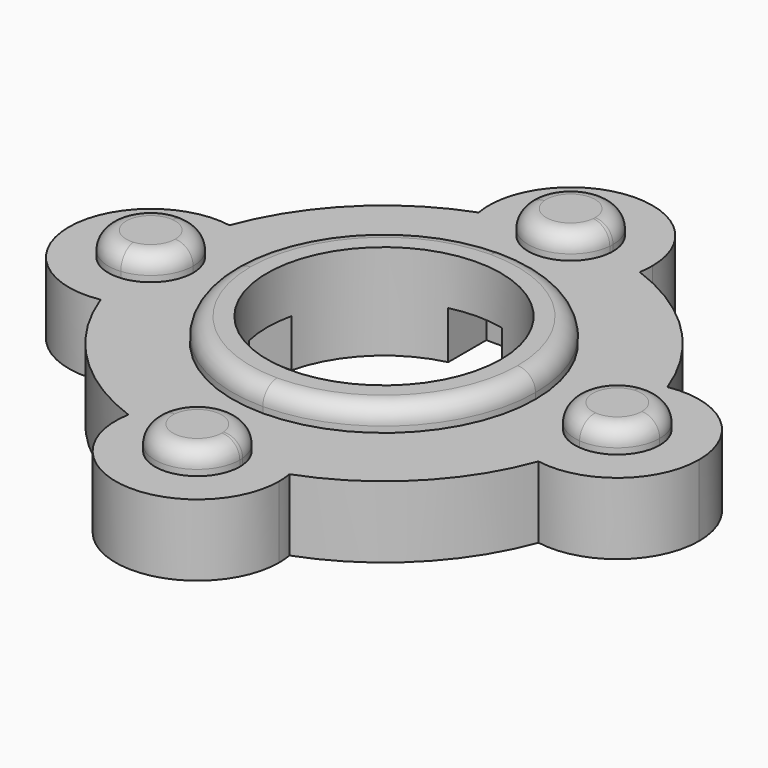
from build123d import *

# Parameters (mm, degrees)
F0_R     = 4.9
F1_DEPTH = 3
F2_DEPTH = 4
F4_DEPTH = 2
F5_R     = 0.75


with BuildPart() as f1:
    # F0 (on Top) → F1 (new body)
    with BuildSketch(Plane.XY):
        with BuildLine():
            ThreePointArc((-9.6173636364, -1.7706376495), (-9.779, 0), (-9.6173636364, 1.7706376495))
            ThreePointArc((-9.6173636364, 1.7706376495), (-11.557, 0), (-9.6173636364, -1.7706376495))
        make_face()
        with BuildLine():
            ThreePointArc((1.778, 9.779), (-0.080901975, 11.5551584587), (-1.7706376495, 9.6173636364))
            ThreePointArc((-1.7706376495, 9.6173636364), (0, 9.779), (1.7706376495, 9.6173636364))
            ThreePointArc((1.7706376495, 9.6173636364), (1.7761584587, 9.698098025), (1.778, 9.779))
        make_face()
        with BuildLine():
            ThreePointArc((-3.3758870855, -9.1778116883), (-2.201881727, -7.1503581719), (0, -6.35))
            ThreePointArc((0, -6.35), (-4.4901280605, -4.4901280605), (-6.35, 0))
            ThreePointArc((-6.35, 0), (-7.1503581719, -2.201881727), (-9.1778116883, -3.3758870855))
            ThreePointArc((-9.1778116883, -3.3758870855), (-6.9147972132, -6.9147972132), (-3.3758870855, -9.1778116883))
        make_face()
        with BuildLine():
            ThreePointArc((-8.001, 0), (-8.4658599742, 1.1987273555), (-9.6173636364, 1.7706376495))
            ThreePointArc((-9.6173636364, 1.7706376495), (-9.779, 0), (-9.6173636364, -1.7706376495))
            ThreePointArc((-9.6173636364, -1.7706376495), (-8.4658599742, -1.1987273555), (-8.001, 0))
        make_face()
        with BuildLine():
            ThreePointArc((3.3758870855, -9.1778116883), (2.201881727, -7.1503581719), (0, -6.35))
            ThreePointArc((0, -6.35), (-2.201881727, -7.1503581719), (-3.3758870855, -9.1778116883))
            ThreePointArc((-3.3758870855, -9.1778116883), (-2.5826305757, -9.4318004808), (-1.7706376495, -9.6173636364))
            ThreePointArc((-1.7706376495, -9.6173636364), (0, -8.001), (1.7706376495, -9.6173636364))
            ThreePointArc((1.7706376495, -9.6173636364), (2.5826305757, -9.4318004808), (3.3758870855, -9.1778116883))
        make_face()
        with BuildLine():
            ThreePointArc((9.1778116883, 3.3758870855), (7.1503581719, 2.201881727), (6.35, 0))
            ThreePointArc((6.35, 0), (7.1503581719, -2.201881727), (9.1778116883, -3.3758870855))
            ThreePointArc((9.1778116883, -3.3758870855), (9.4318004808, -2.5826305757), (9.6173636364, -1.7706376495))
            ThreePointArc((9.6173636364, -1.7706376495), (8.001, 0), (9.6173636364, 1.7706376495))
            ThreePointArc((9.6173636364, 1.7706376495), (9.4318004808, 2.5826305757), (9.1778116883, 3.3758870855))
        make_face()
        with BuildLine():
            ThreePointArc((-9.1778116883, -3.3758870855), (-7.1503581719, -2.201881727), (-6.35, 0))
            ThreePointArc((-6.35, 0), (-7.1503581719, 2.201881727), (-9.1778116883, 3.3758870855))
            ThreePointArc((-9.1778116883, 3.3758870855), (-9.4318004808, 2.5826305757), (-9.6173636364, 1.7706376495))
            ThreePointArc((-9.6173636364, 1.7706376495), (-8.4658599742, 1.1987273555), (-8.001, 0))
            ThreePointArc((-8.001, 0), (-8.4658599742, -1.1987273555), (-9.6173636364, -1.7706376495))
            ThreePointArc((-9.6173636364, -1.7706376495), (-9.4318004808, -2.5826305757), (-9.1778116883, -3.3758870855))
        make_face()
        with BuildLine():
            ThreePointArc((11.557, 0), (10.9777273555, 1.3131400258), (9.6173636364, 1.7706376495))
            ThreePointArc((9.6173636364, 1.7706376495), (9.7385070724, 0.889), (9.779, 0))
            ThreePointArc((9.779, 0), (9.7385070724, -0.889), (9.6173636364, -1.7706376495))
            ThreePointArc((9.6173636364, -1.7706376495), (10.9777273555, -1.3131400258), (11.557, 0))
        make_face()
        with BuildLine():
            ThreePointArc((1.778, -9.779), (1.7761584587, -9.698098025), (1.7706376495, -9.6173636364))
            ThreePointArc((1.7706376495, -9.6173636364), (0, -9.779), (-1.7706376495, -9.6173636364))
            ThreePointArc((-1.7706376495, -9.6173636364), (-0.080901975, -11.5551584587), (1.778, -9.779))
        make_face()
        with BuildLine():
            ThreePointArc((-9.6173636364, 1.7706376495), (-9.4318004808, 2.5826305757), (-9.1778116883, 3.3758870855))
            ThreePointArc((-9.1778116883, 3.3758870855), (-13.208, 0), (-9.1778116883, -3.3758870855))
            ThreePointArc((-9.1778116883, -3.3758870855), (-9.4318004808, -2.5826305757), (-9.6173636364, -1.7706376495))
            ThreePointArc((-9.6173636364, -1.7706376495), (-11.557, 0), (-9.6173636364, 1.7706376495))
        make_face()
        with BuildLine():
            ThreePointArc((1.7706376495, 9.6173636364), (0, 9.779), (-1.7706376495, 9.6173636364))
            ThreePointArc((-1.7706376495, 9.6173636364), (0, 8.001), (1.7706376495, 9.6173636364))
        make_face()
        with BuildLine():
            ThreePointArc((3.429, 9.779), (-0.3017649614, 13.1946959625), (-3.3758870855, 9.1778116883))
            ThreePointArc((-3.3758870855, 9.1778116883), (-2.5826305757, 9.4318004808), (-1.7706376495, 9.6173636364))
            ThreePointArc((-1.7706376495, 9.6173636364), (-0.080901975, 11.5551584587), (1.778, 9.779))
            ThreePointArc((1.778, 9.779), (1.7761584587, 9.698098025), (1.7706376495, 9.6173636364))
            ThreePointArc((1.7706376495, 9.6173636364), (2.5826305757, 9.4318004808), (3.3758870855, 9.1778116883))
            ThreePointArc((3.3758870855, 9.1778116883), (3.4156959625, 9.4772350386), (3.429, 9.779))
        make_face()
        with BuildLine():
            ThreePointArc((13.208, 0), (11.980881727, 2.6286418281), (9.1778116883, 3.3758870855))
            ThreePointArc((9.1778116883, 3.3758870855), (9.4318004808, 2.5826305757), (9.6173636364, 1.7706376495))
            ThreePointArc((9.6173636364, 1.7706376495), (10.9777273555, 1.3131400258), (11.557, 0))
            ThreePointArc((11.557, 0), (10.9777273555, -1.3131400258), (9.6173636364, -1.7706376495))
            ThreePointArc((9.6173636364, -1.7706376495), (9.4318004808, -2.5826305757), (9.1778116883, -3.3758870855))
            ThreePointArc((9.1778116883, -3.3758870855), (11.980881727, -2.6286418281), (13.208, 0))
        make_face()
        with BuildLine():
            ThreePointArc((0, -6.35), (4.4901280605, -4.4901280605), (6.35, 0))
            ThreePointArc((6.35, 0), (4.4901280605, 4.4901280605), (0, 6.35))
            ThreePointArc((0, 6.35), (-4.4901280605, 4.4901280605), (-6.35, 0))
            ThreePointArc((-6.35, 0), (-4.4901280605, -4.4901280605), (0, -6.35))
        make_face()
        Circle(F0_R, mode=Mode.SUBTRACT)
        with BuildLine():
            ThreePointArc((-6.35, 0), (-4.4901280605, 4.4901280605), (0, 6.35))
            ThreePointArc((0, 6.35), (-2.201881727, 7.1503581719), (-3.3758870855, 9.1778116883))
            ThreePointArc((-3.3758870855, 9.1778116883), (-6.9147972132, 6.9147972132), (-9.1778116883, 3.3758870855))
            ThreePointArc((-9.1778116883, 3.3758870855), (-7.1503581719, 2.201881727), (-6.35, 0))
        make_face()
        with BuildLine():
            ThreePointArc((9.1778116883, -3.3758870855), (7.1503581719, -2.201881727), (6.35, 0))
            ThreePointArc((6.35, 0), (4.4901280605, -4.4901280605), (0, -6.35))
            ThreePointArc((0, -6.35), (2.201881727, -7.1503581719), (3.3758870855, -9.1778116883))
            ThreePointArc((3.3758870855, -9.1778116883), (6.9147972132, -6.9147972132), (9.1778116883, -3.3758870855))
        make_face()
        with BuildLine():
            ThreePointArc((0, 6.35), (4.4901280605, 4.4901280605), (6.35, 0))
            ThreePointArc((6.35, 0), (7.1503581719, 2.201881727), (9.1778116883, 3.3758870855))
            ThreePointArc((9.1778116883, 3.3758870855), (6.9147972132, 6.9147972132), (3.3758870855, 9.1778116883))
            ThreePointArc((3.3758870855, 9.1778116883), (2.201881727, 7.1503581719), (0, 6.35))
        make_face()
        with BuildLine():
            ThreePointArc((9.779, 0), (9.7385070724, 0.889), (9.6173636364, 1.7706376495))
            ThreePointArc((9.6173636364, 1.7706376495), (8.001, 0), (9.6173636364, -1.7706376495))
            ThreePointArc((9.6173636364, -1.7706376495), (9.7385070724, -0.889), (9.779, 0))
        make_face()
        with BuildLine():
            ThreePointArc((-1.7706376495, -9.6173636364), (0, -9.779), (1.7706376495, -9.6173636364))
            ThreePointArc((1.7706376495, -9.6173636364), (0, -8.001), (-1.7706376495, -9.6173636364))
        make_face()
        with BuildLine():
            ThreePointArc((-3.3758870855, 9.1778116883), (-2.201881727, 7.1503581719), (0, 6.35))
            ThreePointArc((0, 6.35), (2.201881727, 7.1503581719), (3.3758870855, 9.1778116883))
            ThreePointArc((3.3758870855, 9.1778116883), (2.5826305757, 9.4318004808), (1.7706376495, 9.6173636364))
            ThreePointArc((1.7706376495, 9.6173636364), (0, 8.001), (-1.7706376495, 9.6173636364))
            ThreePointArc((-1.7706376495, 9.6173636364), (-2.5826305757, 9.4318004808), (-3.3758870855, 9.1778116883))
        make_face()
        with BuildLine():
            ThreePointArc((3.429, -9.779), (3.4156959625, -9.4772350386), (3.3758870855, -9.1778116883))
            ThreePointArc((3.3758870855, -9.1778116883), (2.5826305757, -9.4318004808), (1.7706376495, -9.6173636364))
            ThreePointArc((1.7706376495, -9.6173636364), (1.7761584587, -9.698098025), (1.778, -9.779))
            ThreePointArc((1.778, -9.779), (-0.080901975, -11.5551584587), (-1.7706376495, -9.6173636364))
            ThreePointArc((-1.7706376495, -9.6173636364), (-2.5826305757, -9.4318004808), (-3.3758870855, -9.1778116883))
            ThreePointArc((-3.3758870855, -9.1778116883), (-0.3017649614, -13.1946959625), (3.429, -9.779))
        make_face()
    extrude(amount=F1_DEPTH)

    # F0 (on Top) → F2 (join)
    with BuildSketch(Plane.XY):
        with BuildLine():
            ThreePointArc((0, -6.35), (4.4901280605, -4.4901280605), (6.35, 0))
            ThreePointArc((6.35, 0), (4.4901280605, 4.4901280605), (0, 6.35))
            ThreePointArc((0, 6.35), (-4.4901280605, 4.4901280605), (-6.35, 0))
            ThreePointArc((-6.35, 0), (-4.4901280605, -4.4901280605), (0, -6.35))
        make_face()
        Circle(F0_R, mode=Mode.SUBTRACT)
        with BuildLine():
            ThreePointArc((-9.6173636364, -1.7706376495), (-9.779, 0), (-9.6173636364, 1.7706376495))
            ThreePointArc((-9.6173636364, 1.7706376495), (-11.557, 0), (-9.6173636364, -1.7706376495))
        make_face()
        with BuildLine():
            ThreePointArc((-8.001, 0), (-8.4658599742, 1.1987273555), (-9.6173636364, 1.7706376495))
            ThreePointArc((-9.6173636364, 1.7706376495), (-9.779, 0), (-9.6173636364, -1.7706376495))
            ThreePointArc((-9.6173636364, -1.7706376495), (-8.4658599742, -1.1987273555), (-8.001, 0))
        make_face()
        with BuildLine():
            ThreePointArc((1.778, 9.779), (-0.080901975, 11.5551584587), (-1.7706376495, 9.6173636364))
            ThreePointArc((-1.7706376495, 9.6173636364), (0, 9.779), (1.7706376495, 9.6173636364))
            ThreePointArc((1.7706376495, 9.6173636364), (1.7761584587, 9.698098025), (1.778, 9.779))
        make_face()
        with BuildLine():
            ThreePointArc((1.7706376495, 9.6173636364), (0, 9.779), (-1.7706376495, 9.6173636364))
            ThreePointArc((-1.7706376495, 9.6173636364), (0, 8.001), (1.7706376495, 9.6173636364))
        make_face()
        with BuildLine():
            ThreePointArc((11.557, 0), (10.9777273555, 1.3131400258), (9.6173636364, 1.7706376495))
            ThreePointArc((9.6173636364, 1.7706376495), (9.7385070724, 0.889), (9.779, 0))
            ThreePointArc((9.779, 0), (9.7385070724, -0.889), (9.6173636364, -1.7706376495))
            ThreePointArc((9.6173636364, -1.7706376495), (10.9777273555, -1.3131400258), (11.557, 0))
        make_face()
        with BuildLine():
            ThreePointArc((9.779, 0), (9.7385070724, 0.889), (9.6173636364, 1.7706376495))
            ThreePointArc((9.6173636364, 1.7706376495), (8.001, 0), (9.6173636364, -1.7706376495))
            ThreePointArc((9.6173636364, -1.7706376495), (9.7385070724, -0.889), (9.779, 0))
        make_face()
        with BuildLine():
            ThreePointArc((-1.7706376495, -9.6173636364), (0, -9.779), (1.7706376495, -9.6173636364))
            ThreePointArc((1.7706376495, -9.6173636364), (0, -8.001), (-1.7706376495, -9.6173636364))
        make_face()
        with BuildLine():
            ThreePointArc((1.778, -9.779), (1.7761584587, -9.698098025), (1.7706376495, -9.6173636364))
            ThreePointArc((1.7706376495, -9.6173636364), (0, -9.779), (-1.7706376495, -9.6173636364))
            ThreePointArc((-1.7706376495, -9.6173636364), (-0.080901975, -11.5551584587), (1.778, -9.779))
        make_face()
    extrude(amount=F2_DEPTH)

    # F3 (on face) → F4 (cut)
    with BuildSketch(Plane.XY):
        with BuildLine():
            ThreePointArc((-1.125, 4.7691063104), (0, 4.9), (1.125, 4.7691063104))
            Line((1.125, 4.7691063104), (1.125, 6.7691063104))
            Line((1.125, 6.7691063104), (-1.125, 6.7691063104))
            Line((-1.125, 6.7691063104), (-1.125, 4.7691063104))
        make_face()
        with BuildLine():
            Line((6.7691063104, 1.125), (4.7691063104, 1.125))
            ThreePointArc((4.7691063104, 1.125), (4.8671665741, 0.5662945695), (4.9, 0))
            ThreePointArc((4.9, 0), (4.8671665741, -0.5662945695), (4.7691063104, -1.125))
            Line((4.7691063104, -1.125), (6.7691063104, -1.125))
            Line((6.7691063104, -1.125), (6.7691063104, 1.125))
        make_face()
        with BuildLine():
            Line((1.125, -6.7691063104), (1.125, -4.7691063104))
            ThreePointArc((1.125, -4.7691063104), (0, -4.9), (-1.125, -4.7691063104))
            Line((-1.125, -4.7691063104), (-1.125, -6.7691063104))
            Line((-1.125, -6.7691063104), (1.125, -6.7691063104))
        make_face()
        with BuildLine():
            ThreePointArc((-4.7691063104, -1.125), (-4.9, 0), (-4.7691063104, 1.125))
            Line((-4.7691063104, 1.125), (-6.7691063104, 1.125))
            Line((-6.7691063104, 1.125), (-6.7691063104, -1.125))
            Line((-6.7691063104, -1.125), (-4.7691063104, -1.125))
        make_face()
    extrude(amount=F4_DEPTH, mode=Mode.SUBTRACT)

    # F5
    f5_edges = [f1.edges().sort_by_distance(p)[0] for p in [
        (-9.940636, 1.770638, 4),
        (1.770638, 9.940636, 4),
        (9.940636, -1.770638, 4),
        (1.770638, -9.940636, 4),
        (0, -6.35, 4),
    ]]
    fillet(f5_edges, radius=F5_R)


solid = f1.part
